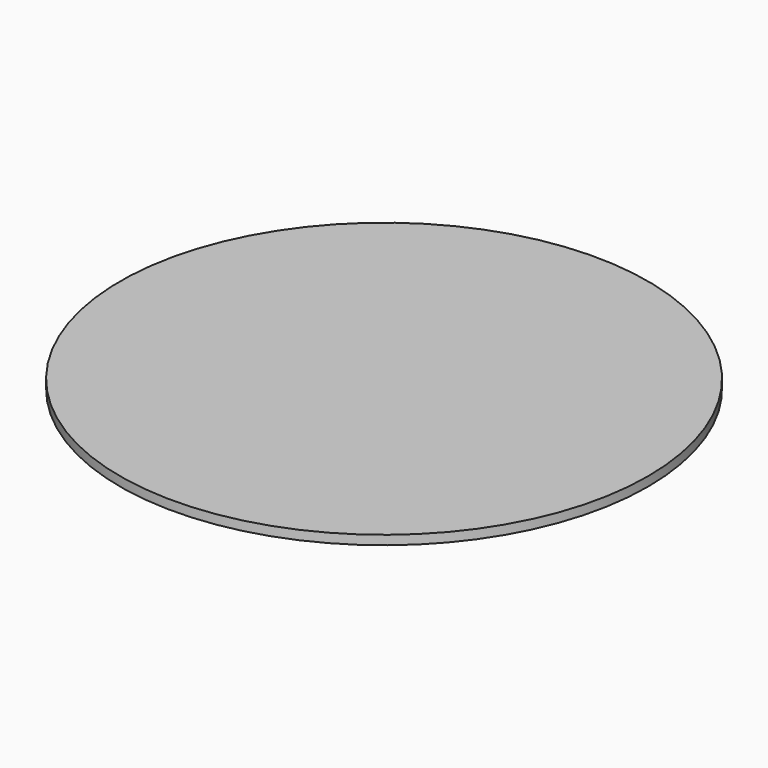
from build123d import *

# Parameters (mm, degrees)
F0_R     = 72.9648324798
F1_DEPTH = 2.54


# Not quite as in the source:
# - the program builds the solid bodies; features that only make, move or delete a surface that nothing else refers to are left out


with BuildPart() as f1:
    # F0 (on Top) → F1 (new body)
    with BuildSketch(Plane.XY):
        Circle(F0_R)
    extrude(amount=F1_DEPTH)


solid = f1.part
